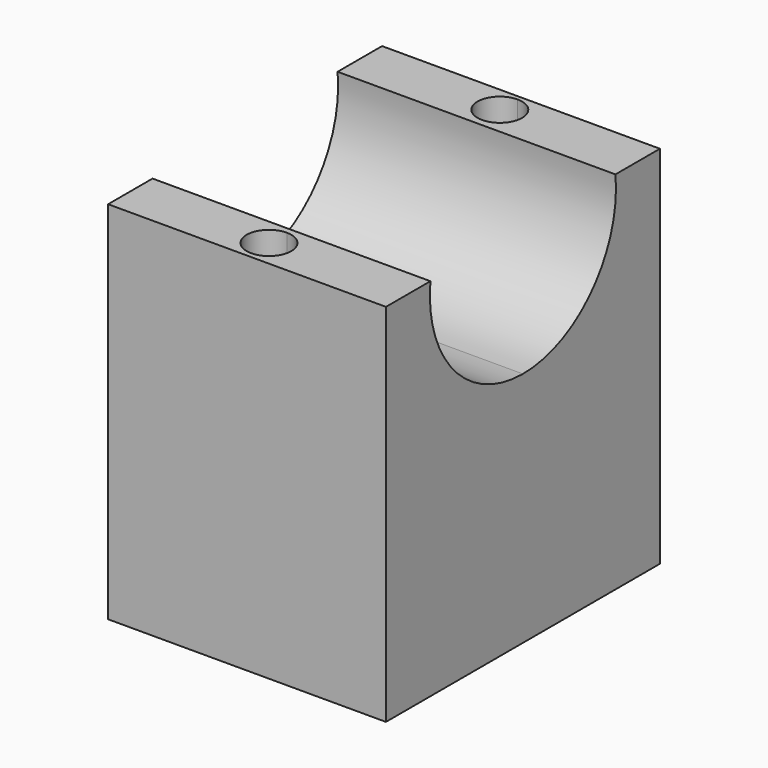
from build123d import *

# Parameters (mm, degrees)
F1_DEPTH = 20
F3_DEPTH = 20


with BuildPart() as f1:
    # F0 (on Right) → F1 (new body)
    with BuildSketch(Plane.YZ):
        with BuildLine():
            ThreePointArc((0.551975, -0.016701), (-5.674131, 2.758224), (-7.773025, 9.243533))
            Line((-7.773025, 9.243533), (-11.773025, 9.243533))
            Line((-11.773025, 9.243533), (-11.773025, -17.058467))
            Line((-11.773025, -17.058467), (0.551975, -17.058467))
            Line((0.551975, -17.058467), (0.551975, -0.016701))
        make_face()
        with BuildLine():
            ThreePointArc((8.876975, 9.243533), (6.77808, 2.758224), (0.551975, -0.016701))
            Line((0.551975, -0.016701), (0.551975, -17.058467))
            Line((0.551975, -17.058467), (12.876975, -17.058467))
            Line((12.876975, -17.058467), (12.876975, 9.243533))
            Line((12.876975, 9.243533), (8.876975, 9.243533))
        make_face()
    extrude(amount=F1_DEPTH)

    # F2 (on Top) → F3 (cut, symmetric)
    with BuildSketch(Plane.XY):
        with BuildLine():
            Line((10.007922, -8.205494), (10.007922, -9.805494))
            Line((10.007922, -9.805494), (10.007922, -9.905494))
            Line((10.007922, -9.905494), (10.007922, -11.405494))
            ThreePointArc((10.007922, -11.405494), (11.139292, -10.936865), (11.607922, -9.805494))
            ThreePointArc((11.607922, -9.805494), (11.139292, -8.674123), (10.007922, -8.205494))
        make_face()
        with BuildLine():
            Line((10.007922, -9.905494), (10.007922, -9.805494))
            Line((10.007922, -9.805494), (10.007922, -8.205494))
            ThreePointArc((10.007922, -8.205494), (8.407922, -9.805494), (10.007922, -11.405494))
            Line((10.007922, -11.405494), (10.007922, -9.905494))
        make_face()
        with BuildLine():
            ThreePointArc((10.007922, 12.564938), (8.407922, 10.964938), (10.007922, 9.364938))
            Line((10.007922, 9.364938), (10.007922, 10.864938))
            Line((10.007922, 10.864938), (10.007922, 10.964938))
            Line((10.007922, 10.964938), (10.007922, 12.564938))
        make_face()
        with BuildLine():
            Line((10.007922, 10.864938), (10.007922, 9.364938))
            ThreePointArc((10.007922, 9.364938), (11.139292, 9.833568), (11.607922, 10.964938))
            ThreePointArc((11.607922, 10.964938), (11.139292, 12.096309), (10.007922, 12.564938))
            Line((10.007922, 12.564938), (10.007922, 10.964938))
            Line((10.007922, 10.964938), (10.007922, 10.864938))
        make_face()
    extrude(amount=F3_DEPTH, both=True, mode=Mode.SUBTRACT)


solid = f1.part
